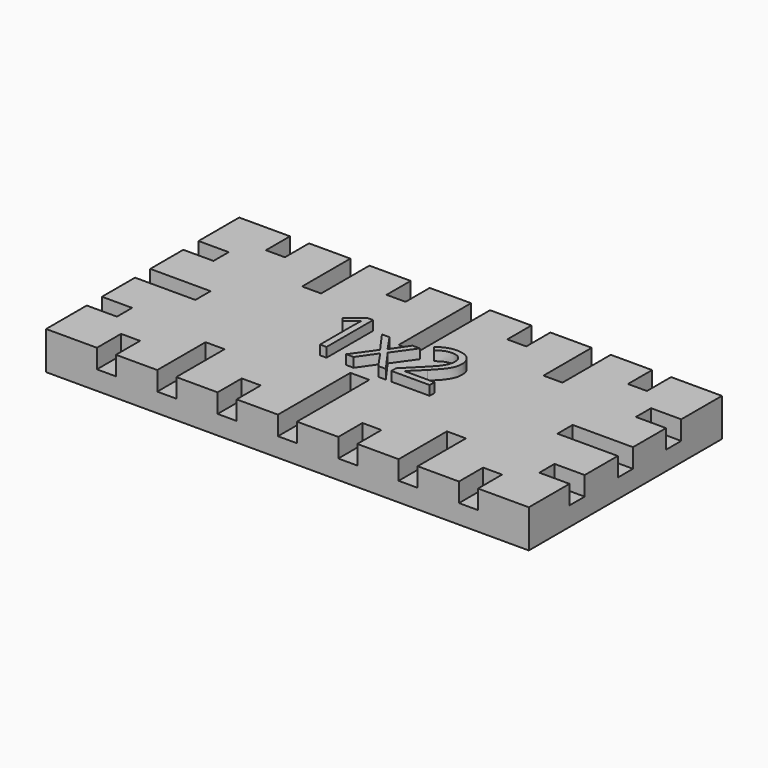
from build123d import *

# Parameters (mm, degrees)
F0_W         = 50.8
F0_H         = 25.4
F1_DEPTH     = 4
F2_W         = 2
F2_H         = 19.05
F2_H_2       = 6.35
F2_W_2       = 12.7
F2_H_3       = 2
F2_W_3       = 6.35
F2_H_4       = 12.7
F3_DEPTH     = 2
F4_TEXT_SIZE = 8.5848202515
F5_DEPTH     = 1


# Not quite as in the source:
# - Text() gives the source's letters only with a copy of the font that has no kerning and outlines rounded to 1/6400 em; it was checked with that copy


with BuildPart() as f1:
    # F0 (on Top) → F1 (new body)
    with BuildSketch(Plane.XY):
        Rectangle(F0_W, F0_H)
    extrude(amount=F1_DEPTH)

    # F2 (on face) → F3 (cut)
    with BuildSketch(Plane.XY.offset(4)):
        with Locations((0, -12.7)):
            Rectangle(F2_W, F2_H)
        with Locations((6.35, -12.7)):
            Rectangle(F2_W, F2_H_2)
        with Locations((-6.35, -12.7)):
            Rectangle(F2_W, F2_H_2)
        with Locations((-25.4, 0)):
            Rectangle(F2_W_2, F2_H_3)
        with Locations((-25.4, 6.35)):
            Rectangle(F2_W_3, F2_H_3)
        with Locations((-25.4, -6.35)):
            Rectangle(F2_W_3, F2_H_3)
        with Locations((0, 12.7)):
            Rectangle(F2_W, F2_H)
        with Locations((-6.35, 12.7)):
            Rectangle(F2_W, F2_H_2)
        with Locations((6.35, 12.7)):
            Rectangle(F2_W, F2_H_2)
        with Locations((25.4, 0)):
            Rectangle(F2_W_2, F2_H_3)
        with Locations((25.4, -6.35)):
            Rectangle(F2_W_3, F2_H_3)
        with Locations((25.4, 6.35)):
            Rectangle(F2_W_3, F2_H_3)
        with Locations((-12.7, 12.7000001177)):
            Rectangle(F2_W, F2_H_4)
        with Locations((-19.05, 12.7000001177)):
            Rectangle(F2_W, F2_H_2)
        with Locations((-12.7, -12.7000005066)):
            Rectangle(F2_W, F2_H_4)
        with Locations((-19.05, -12.7000005066)):
            Rectangle(F2_W, F2_H_2)
        with Locations((12.700000225, -12.7)):
            Rectangle(F2_W, F2_H_4)
        with Locations((19.050000225, -12.7)):
            Rectangle(F2_W, F2_H_2)
        with Locations((12.700000225, 12.7)):
            Rectangle(F2_W, F2_H_4)
        with Locations((19.050000225, 12.7)):
            Rectangle(F2_W, F2_H_2)
    extrude(amount=-F3_DEPTH, mode=Mode.SUBTRACT)


with BuildPart() as f5:
    # F4 (on face) → F5 (new body)
    with BuildSketch(Plane.XY.offset(4)):
        with Locations((-7.2052128095, -2.302775858)):
            Text('1x2', F4_TEXT_SIZE, font='Open Sans', text_align=(TextAlign.LEFT, TextAlign.BOTTOM))
    extrude(amount=F5_DEPTH)


solid = Compound([f1.part, f5.part])
